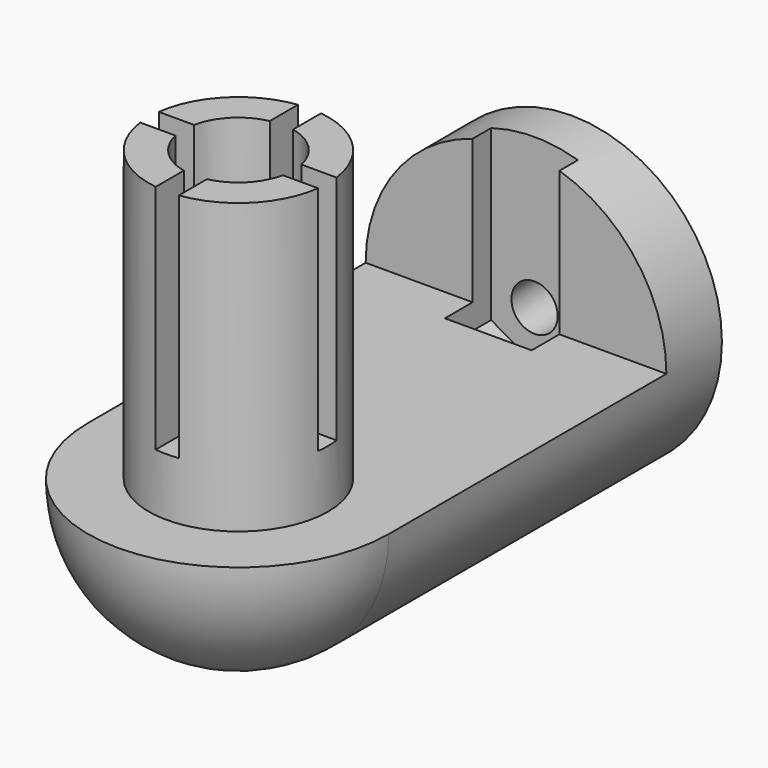
from build123d import *
from build123d import SkipClean  # not in build123d's __all__

# Parameters (mm, degrees)
F1_ANGLE  = 180
F2_R      = 13
F3_DEPTH  = 6
F4_R      = 2
F5_DEPTH  = 6
F7_DEPTH  = 2
F8_DEPTH  = 5
F9_DEPTH  = 3
F10_W     = 7.5
F10_H     = 12.1405349095
F11_DEPTH = 2
F12_R     = 2.8
F12_R_2   = 2
F13_DEPTH = 1.8
F14_R     = 3.3
F15_DEPTH = 25
F17_R     = 4.9
F18_DEPTH = 7.3
F19_DEPTH = 25
F20_R     = 7.75
F20_R_2   = 3.3
F21_DEPTH = 25
F23_DEPTH = 20


# Not quite as in the source:
# - after a boolean that leaves OpenCascade's solid faulty, fix() repairs it


with BuildPart() as f1:
    # F0 (on Top) → F1 (revolve)
    with BuildSketch(Plane.XY):
        with BuildLine():
            Line((13, 0), (0, 0))
            Line((0, 0), (0, -43))
            ThreePointArc((0, -43), (9.1923881554, -39.1923881554), (13, -30))
            Line((13, -30), (13, 0))
        make_face()
    revolve(axis=Axis((0, -21.5, 0), (0, 1, 0)), revolution_arc=F1_ANGLE)

    # F2 (on face) → F3 (join)
    with BuildSketch(Plane(origin=(0, 0, 0), x_dir=(-1, 0, 0), z_dir=(0, 1, 0))):
        Circle(F2_R)
    with SkipClean():  # cleaning this boolean's faces spoils the solid; the shape is the same uncleaned
        extrude(amount=F3_DEPTH)

    # F4 (on face) → F5 (cut)
    with BuildSketch(Plane(origin=(0, 6, 0), x_dir=(-1, 0, 0), z_dir=(0, 1, 0))):
        Circle(F4_R)
    extrude(amount=-F5_DEPTH, mode=Mode.SUBTRACT)

    add(f1.part.fix(), mode=Mode.REPLACE)

    # F6 (on face) → F7 (cut)
    with BuildSketch(Plane(origin=(0, 0, 0), x_dir=(-1, 0, 0), z_dir=(0, 1, 0))):
        Polygon((3.75, 2.1650635095), (0, 4.3301270189), (-3.75, 2.1650635095), (-3.75, -2.1650635095), (0, -4.3301270189), (3.75, -2.1650635095), align=None)
    extrude(amount=F7_DEPTH, mode=Mode.SUBTRACT)

    # F8 (cut): a face of the model
    f8_faces = [f1.faces().sort_by_distance(p)[0] for p in [
        (-3.6354356076, 2, 0),
    ]]
    extrude(f8_faces, amount=F8_DEPTH, mode=Mode.SUBTRACT)

    # F9 (cut): a face of the model
    f9_faces = [f1.faces().sort_by_distance(p)[0] for p in [
        (0, 0, -0.8488263632),
    ]]
    extrude(f9_faces, amount=-F9_DEPTH, mode=Mode.SUBTRACT)

    # F10 (on face) → F11 (cut)
    with BuildSketch(Plane.XZ):
        with Locations((0, 8.2353309642)):
            Rectangle(F10_W, F10_H)
    extrude(amount=-F11_DEPTH, mode=Mode.SUBTRACT)

    # F12 (on face) → F13 (join)
    with BuildSketch(Plane(origin=(0, 6, 0), x_dir=(-1, 0, 0), z_dir=(0, 1, 0))):
        Circle(F12_R)
        Circle(F12_R_2, mode=Mode.SUBTRACT)
    extrude(amount=F13_DEPTH)

    # F14 (on face) → F15 (cut)
    with BuildSketch(Plane.XY):
        with Locations((0, -30)):
            Circle(F14_R)
    extrude(amount=-F15_DEPTH, mode=Mode.SUBTRACT)

    # F17 (on face) → F18 (cut)
    with BuildSketch(Plane.XY.offset(-12.5741798937)):
        with Locations((0, -30)):
            Circle(F17_R)
    extrude(amount=F18_DEPTH, mode=Mode.SUBTRACT)

    # F19 (cut): a face of the model
    f19_faces = [f1.faces().sort_by_distance(p)[0] for p in [
        (-4.7614070709, -30, -5.2741798937),
    ]]
    extrude(f19_faces, amount=F19_DEPTH, mode=Mode.SUBTRACT)

    # F20 (on face) → F21 (join)
    with BuildSketch(Plane.XY):
        with Locations((0, -30)):
            Circle(F20_R)
        with Locations((0, -30)):
            Circle(F20_R_2, mode=Mode.SUBTRACT)
    extrude(amount=F21_DEPTH)

    # F22 (on face) → F23 (cut)
    with BuildSketch(Plane.XY.offset(25)):
        with BuildLine():
            ThreePointArc((4.6435439053, -31), (4.7233109971, -30.502825243), (4.75, -30))
            ThreePointArc((4.75, -30), (4.7233109971, -29.497174757), (4.6435439053, -29))
            Line((4.6435439053, -29), (1, -29))
            Line((1, -29), (1, -31))
            Line((1, -31), (4.6435439053, -31))
        make_face()
        with BuildLine():
            ThreePointArc((4.6435439053, -29), (4.7233109971, -29.497174757), (4.75, -30))
            ThreePointArc((4.75, -30), (4.7233109971, -30.502825243), (4.6435439053, -31))
            Line((4.6435439053, -31), (10.7483885819, -31))
            Line((10.7483885819, -31), (10.7483885819, -29))
            Line((10.7483885819, -29), (4.6435439053, -29))
        make_face()
        with BuildLine():
            Line((1, -29), (4.6435439053, -29))
            ThreePointArc((4.6435439053, -29), (3.3587572106, -26.6412427894), (1, -25.3564560947))
            Line((1, -25.3564560947), (1, -29))
        make_face()
        with BuildLine():
            ThreePointArc((1, -34.6435439053), (3.3587572106, -33.3587572106), (4.6435439053, -31))
            Line((4.6435439053, -31), (1, -31))
            Line((1, -31), (1, -34.6435439053))
        make_face()
        with BuildLine():
            Line((1, -29), (1, -25.3564560947))
            ThreePointArc((1, -25.3564560947), (0, -25.25), (-1, -25.3564560947))
            Line((-1, -25.3564560947), (-1, -29))
            Line((-1, -29), (1, -29))
        make_face()
        with BuildLine():
            ThreePointArc((-1, -25.3564560947), (0, -25.25), (1, -25.3564560947))
            Line((1, -25.3564560947), (1, -19.8912940045))
            Line((1, -19.8912940045), (-1, -19.8912940045))
            Line((-1, -19.8912940045), (-1, -25.3564560947))
        make_face()
        with BuildLine():
            Line((1, -40.1087059955), (1, -34.6435439053))
            ThreePointArc((1, -34.6435439053), (0, -34.75), (-1, -34.6435439053))
            Line((-1, -34.6435439053), (-1, -40.1087059955))
            Line((-1, -40.1087059955), (1, -40.1087059955))
        make_face()
        with BuildLine():
            ThreePointArc((-1, -34.6435439053), (0, -34.75), (1, -34.6435439053))
            Line((1, -34.6435439053), (1, -31))
            Line((1, -31), (-1, -31))
            Line((-1, -31), (-1, -34.6435439053))
        make_face()
        with BuildLine():
            Line((-1, -29), (-1, -25.3564560947))
            ThreePointArc((-1, -25.3564560947), (-3.3587572106, -26.6412427894), (-4.6435439053, -29))
            Line((-4.6435439053, -29), (-1, -29))
        make_face()
        with BuildLine():
            Line((-1, -31), (-1, -29))
            Line((-1, -29), (-4.6435439053, -29))
            ThreePointArc((-4.6435439053, -29), (-4.75, -30), (-4.6435439053, -31))
            Line((-4.6435439053, -31), (-1, -31))
        make_face()
        with BuildLine():
            ThreePointArc((-4.6435439053, -31), (-3.3587572106, -33.3587572106), (-1, -34.6435439053))
            Line((-1, -34.6435439053), (-1, -31))
            Line((-1, -31), (-4.6435439053, -31))
        make_face()
        with BuildLine():
            ThreePointArc((-4.6435439053, -31), (-4.75, -30), (-4.6435439053, -29))
            Line((-4.6435439053, -29), (-10.7483885819, -29))
            Line((-10.7483885819, -29), (-10.7483885819, -31))
            Line((-10.7483885819, -31), (-4.6435439053, -31))
        make_face()
    extrude(amount=-F23_DEPTH, mode=Mode.SUBTRACT)


solid = f1.part
